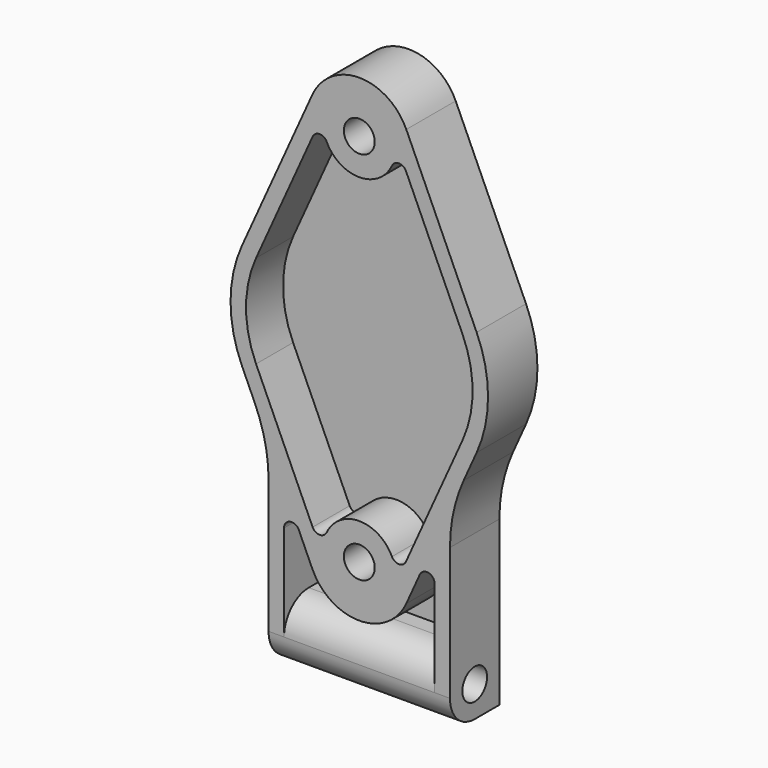
from build123d import *

# Parameters (mm, degrees)
F0_R     = 2
F1_DEPTH = 8
F2_DEPTH = 2
F3_R     = 20
F4_R     = 1
F6_D     = 4
F7_R     = 3.99999


# Not quite as in the source:
# - a fillet or chamfer is up to 0.001 mm smaller than in the source, because OpenCascade refuses the exact size
# - a feature names something its author has since deleted; it is built from what else it names


with BuildPart() as f1:
    # F0 (on Front) → F1 (new body)
    with BuildSketch(Plane.XZ):
        with BuildLine():
            Line((15.1970139668, 6.8636525628), (6.0880650012, 27.0320429916))
            ThreePointArc((6.0880650012, 27.0320429916), (0, 30.9626), (-6.0880650012, 27.0320429916))
            Line((-6.0880650012, 27.0320429916), (-15.1970139668, 6.8636525628))
            ThreePointArc((-15.1970139668, 6.8636525628), (-16.6751, 0), (-15.1970139668, -6.8636525628))
            Line((-15.1970139668, -6.8636525628), (-11.75, -14.4957870449))
            Line((-11.75, -14.4957870449), (-9.75, -18.9240455641))
            Line((-9.75, -18.9240455641), (-6.0880650012, -27.0320429916))
            ThreePointArc((-6.0880650012, -27.0320429916), (0, -30.9626), (6.0880650012, -27.0320429916))
            Line((6.0880650012, -27.0320429916), (9.75, -18.9240455641))
            Line((9.75, -18.9240455641), (11.75, -14.4957870449))
            Line((11.75, -14.4957870449), (15.1970139668, -6.8636525628))
            ThreePointArc((15.1970139668, -6.8636525628), (16.6751, 0), (15.1970139668, 6.8636525628))
        make_face()
        with Locations((0, -24.2824)):
            Circle(F0_R, mode=Mode.SUBTRACT)
        with BuildLine():
            Line((-13.3742945868, 6.0404308054), (-6.0462846285, 22.2655920687))
            ThreePointArc((-6.0462846285, 22.2655920687), (-5.1436901116, 22.8539427752), (-4.2309206889, 22.2815046593))
            ThreePointArc((-4.2309206889, 22.2815046593), (0, 19.6022), (4.2309206889, 22.2815046593))
            ThreePointArc((4.2309206889, 22.2815046593), (5.1436901116, 22.8539427752), (6.0462846285, 22.2655920687))
            Line((6.0462846285, 22.2655920687), (13.3742945868, 6.0404308054))
            ThreePointArc((13.3742945868, 6.0404308054), (14.6751, 0), (13.3742945868, -6.0404308054))
            Line((13.3742945868, -6.0404308054), (6.0462846285, -22.2655920687))
            ThreePointArc((6.0462846285, -22.2655920687), (5.1436901116, -22.8539427752), (4.2309206889, -22.2815046593))
            ThreePointArc((4.2309206889, -22.2815046593), (0, -19.6022), (-4.2309206889, -22.2815046593))
            ThreePointArc((-4.2309206889, -22.2815046593), (-5.1436901116, -22.8539427752), (-6.0462846285, -22.2655920687))
            Line((-6.0462846285, -22.2655920687), (-13.3742945868, -6.0404308054))
            ThreePointArc((-13.3742945868, -6.0404308054), (-14.6751, 0), (-13.3742945868, 6.0404308054))
        make_face(mode=Mode.SUBTRACT)
        with Locations((0, 24.2824)):
            Circle(F0_R, mode=Mode.SUBTRACT)
        Polygon((11.75, -40), (11.75, -14.4957870449), (9.75, -18.9240455641), (9.75, -32), (-9.75, -32), (-9.75, -18.9240455641), (-11.75, -14.4957870449), (-11.75, -40), align=None)
    extrude(amount=F1_DEPTH)

    # F0 (on Front) → F2 (join)
    with BuildSketch(Plane.XZ):
        with BuildLine():
            ThreePointArc((-4.2309206889, 22.2815046593), (-5.1436901116, 22.8539427752), (-6.0462846285, 22.2655920687))
            Line((-6.0462846285, 22.2655920687), (-13.3742945868, 6.0404308054))
            ThreePointArc((-13.3742945868, 6.0404308054), (-14.6751, 0), (-13.3742945868, -6.0404308054))
            Line((-13.3742945868, -6.0404308054), (-6.0462846285, -22.2655920687))
            ThreePointArc((-6.0462846285, -22.2655920687), (-5.1436901116, -22.8539427752), (-4.2309206889, -22.2815046593))
            ThreePointArc((-4.2309206889, -22.2815046593), (0, -19.6022), (4.2309206889, -22.2815046593))
            ThreePointArc((4.2309206889, -22.2815046593), (5.1436901116, -22.8539427752), (6.0462846285, -22.2655920687))
            Line((6.0462846285, -22.2655920687), (13.3742945868, -6.0404308054))
            ThreePointArc((13.3742945868, -6.0404308054), (14.6751, 0), (13.3742945868, 6.0404308054))
            Line((13.3742945868, 6.0404308054), (6.0462846285, 22.2655920687))
            ThreePointArc((6.0462846285, 22.2655920687), (5.1436901116, 22.8539427752), (4.2309206889, 22.2815046593))
            ThreePointArc((4.2309206889, 22.2815046593), (0, 19.6022), (-4.2309206889, 22.2815046593))
        make_face()
        with BuildLine():
            Line((9.75, -32), (9.75, -18.9240455641))
            Line((9.75, -18.9240455641), (6.0880650012, -27.0320429916))
            ThreePointArc((6.0880650012, -27.0320429916), (0, -30.9626), (-6.0880650012, -27.0320429916))
            Line((-6.0880650012, -27.0320429916), (-9.75, -18.9240455641))
            Line((-9.75, -18.9240455641), (-9.75, -32))
            Line((-9.75, -32), (9.75, -32))
        make_face()
    extrude(amount=F2_DEPTH)

    # F3
    f3_edges = [f1.edges().sort_by_distance(p)[0] for p in [
        (11.75, -4, -14.495787),
        (-11.75, -4, -14.495787),
    ]]
    fillet(f3_edges, radius=F3_R)

    # F4
    f4_edges = [f1.edges().sort_by_distance(p)[0] for p in [
        (9.75, -5, -18.924046),
        (-9.75, -5, -18.924046),
    ]]
    fillet(f4_edges, radius=F4_R)

    # F6 (through all)
    with Locations(Plane.YZ.offset(11.75)):
        with Locations((-4, -36)):
            Hole(F6_D / 2)

    # F7 (radius 4 in the source; OpenCascade refuses exactly that, so slightly less here)
    f7_edges = [f1.edges().sort_by_distance(p)[0] for p in [
        (0, -8, -40),
        (0, -8, -32),
    ]]
    fillet(f7_edges, radius=F7_R)


solid = f1.part
